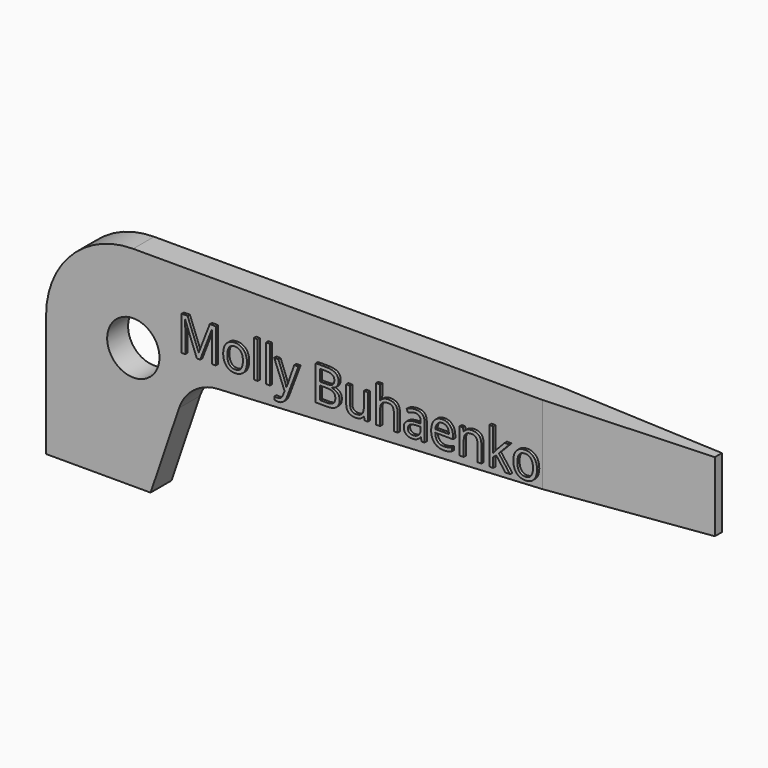
from build123d import *

# Parameters (mm, degrees)
F1_DEPTH     = 2.38125
F2_R         = 2.38125
F3_DEPTH     = 25.4
F5_DEPTH     = 25.4
F6_DEPTH     = 50.8
F7_TEXT_SIZE = 4.4030395957
F8_DEPTH     = 0.254


# Not quite as in the source:
# - Text() gives the source's letters only with a copy of the font that has no kerning and outlines rounded to 1/6400 em; it was checked with that copy


with BuildPart() as f1:
    # F0 (on Front) → F1 (new body)
    with BuildSketch(Plane.XZ):
        with BuildLine():
            Line((60.325, 19.05), (7.9375, 19.05))
            ThreePointArc((7.9375, 19.05), (2.3248399243, 16.7251600757), (0, 11.1125))
            Line((0, 11.1125), (0, 0))
            Line((0, 0), (9.525, 0))
            Line((9.525, 0), (12.1173647876, 7.6271664624))
            ThreePointArc((12.1173647876, 7.6271664624), (13.4786145605, 9.5135918491), (15.6631963617, 10.3130942181))
            Line((15.6631963617, 10.3130942181), (60.325, 12.7))
            Line((60.325, 12.7), (60.325, 19.05))
        make_face()
    extrude(amount=F1_DEPTH)

    # F2 (on face) → F3 (cut)
    with BuildSketch(Plane.XZ.offset(2.38125)):
        with Locations((7.9502, 11.0998)):
            Circle(F2_R)
    extrude(amount=-F3_DEPTH, mode=Mode.SUBTRACT)

    # F4 (on face) → F5 (join)
    with BuildSketch(Plane.XY.offset(19.05)):
        Polygon((60.325, -2.38125), (60.325, -1.59385), (45.2374, -2.38125), align=None)
        Polygon((60.325, 0), (45.2374, 0), (60.325, -0.7874), align=None)
    extrude(amount=F5_DEPTH)

    # F6 (cut): faces of the model
    f6_faces = [f1.faces().sort_by_distance(p)[0] for p in [
        (55.2958, -2.1187833333, 44.45),
        (55.2958, -0.2624666667, 44.45),
    ]]
    extrude(f6_faces, amount=-F6_DEPTH, mode=Mode.SUBTRACT)

    # F7 (on face) → F8 (join)
    with BuildSketch(Plane.XZ.offset(2.38125)):
        with Locations((12.1244783155, 12.3016405851)):
            Text('Molly Buhaenko', F7_TEXT_SIZE, font='Open Sans', text_align=(TextAlign.LEFT, TextAlign.BOTTOM))
    extrude(amount=F8_DEPTH)


solid = f1.part
